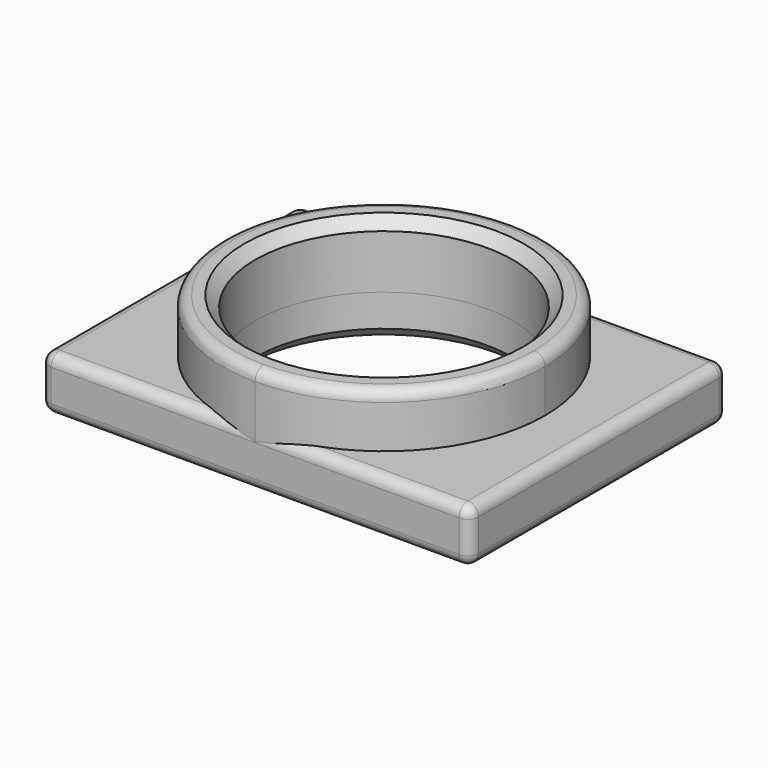
from build123d import *

# Parameters (mm, degrees)
F0_R      = 60
F1_DEPTH  = 50
F2_DEPTH  = 25
F3_R      = 5
F3_2_R    = 5
F4_SIZE   = 5
F4_2_SIZE = 5


with BuildPart() as f1:
    # F0 (on Top) → F1 (new body)
    with BuildSketch(Plane.XY):
        with BuildLine():
            ThreePointArc((-3.096e-07, -75), (53.0330084795, -53.0330086984), (75, 0))
            ThreePointArc((75, 0), (53.0330084621, 53.0330087158), (-3.588e-07, 75))
            ThreePointArc((-3.588e-07, 75), (-75, -2.46e-08), (-3.096e-07, -75))
        make_face()
        Circle(F0_R, mode=Mode.SUBTRACT)
    extrude(amount=F1_DEPTH)

    # F3
    f3_edges = [f1.edges().sort_by_distance(p)[0] for p in [
        (0, -75, 0),
        (0, 75, 25),
        (0, -75, 50),
    ]]
    fillet(f3_edges, radius=F3_R)

    # F4#2
    f4_2_edges = [f1.edges().sort_by_distance(p)[0] for p in [
        (-60, 0, 0),
        (60, 0, 25),
        (-60, 0, 50),
    ]]
    chamfer(f4_2_edges, length=F4_2_SIZE)


with BuildPart() as f2:
    # F0 (on Top) → F2 (new body)
    with BuildSketch(Plane.XY):
        with BuildLine():
            ThreePointArc((-3.096e-07, -75), (53.0330084795, -53.0330086984), (75, 0))
            ThreePointArc((75, 0), (53.0330084621, 53.0330087158), (-3.588e-07, 75))
            ThreePointArc((-3.588e-07, 75), (-75, -2.46e-08), (-3.096e-07, -75))
        make_face()
        Circle(F0_R, mode=Mode.SUBTRACT)
        with BuildLine():
            ThreePointArc((-3.588e-07, 75), (53.0330084621, 53.0330087158), (75, 0))
            ThreePointArc((75, 0), (53.0330084795, -53.0330086984), (-3.096e-07, -75))
            Line((-3.096e-07, -75), (100, -75))
            Line((100, -75), (100, 75))
            Line((100, 75), (-3.588e-07, 75))
        make_face()
        with BuildLine():
            ThreePointArc((-3.096e-07, -75), (-75, -2.46e-08), (-3.588e-07, 75))
            Line((-3.588e-07, 75), (-100, 75))
            Line((-100, 75), (-100, -75))
            Line((-100, -75), (-3.096e-07, -75))
        make_face()
    extrude(amount=F2_DEPTH)

    # F3#2
    f3_2_edges = [f2.edges().sort_by_distance(p)[0] for p in [
        (0, -75, 0),
        (0, 75, 25),
        (100, 0, 25),
        (-100, 0, 25),
        (0, -75, 25),
        (-60, 0, 25),
        (-100, 75, 12.5),
        (-100, -75, 12.5),
        (-100, 0, 0),
        (100, 75, 12.5),
        (0, 75, 0),
        (100, -75, 12.5),
        (100, 0, 0),
    ]]
    fillet(f3_2_edges, radius=F3_2_R)

    # F4
    f4_edges = [f2.edges().sort_by_distance(p)[0] for p in [
        (-60, 0, 0),
    ]]
    chamfer(f4_edges, length=F4_SIZE)


solid = Compound([f1.part, f2.part])
